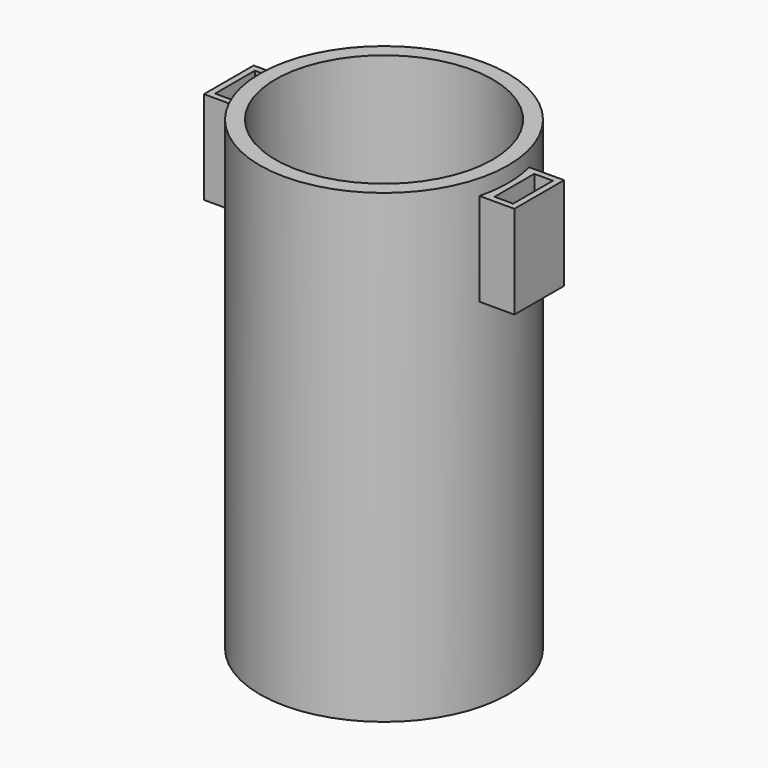
from build123d import *

# Parameters (mm, degrees)
F0_W          = 50.8
F0_H          = 50.8
F1_DEPTH      = 95.25
F3_DEPTH      = 6.35
F5_W          = 3.81
F5_H          = 10.16
F6_DEPTH      = 25.4
F7_T4_DEPTH   = 222.25
F7_T10_DEPTH  = 222.25
F7_T16_DEPTH  = 222.25
F7_T23_DEPTH  = 222.25
F7_T29_DEPTH  = 222.25
F7_T35_DEPTH  = 222.25
F7_T41_DEPTH  = 222.25
F7_T47_DEPTH  = 222.25
F7_T54_DEPTH  = 222.25
F7_T60_DEPTH  = 222.25
F7_T66_DEPTH  = 222.25
F7_T72_DEPTH  = 222.25
F7_T78_DEPTH  = 222.25
F7_T85_DEPTH  = 222.25
F7_T91_DEPTH  = 222.25
F7_T97_DEPTH  = 222.25
F7_T103_DEPTH = 222.25
F7_T109_DEPTH = 222.25
F7_T116_DEPTH = 222.25
F7_T122_DEPTH = 222.25
F8_R          = 22.225
F9_DEPTH      = 88.9


# Not quite as in the source:
# - a fillet or chamfer that OpenCascade refuses, or shapes differently, is made with other operations: its cross-section is extruded or revolved along the edge and cut away or added


with BuildPart() as f1:
    # F0 (on Top) → F1 (new body)
    with BuildSketch(Plane.XY):
        Rectangle(F0_W, F0_H)
    extrude(amount=F1_DEPTH)

    # F2 (on face) → F3 (join)
    with BuildSketch(Plane(origin=(-25.4, 0, 0), x_dir=(0, -1, 0), z_dir=(-1, 0, 0))):
        Polygon((-6.35, 73.025), (6.35, 73.025), (6.35, 92.075), (0, 92.075), (-6.35, 92.075), align=None)
    extrude(amount=F3_DEPTH)

    # F4: F1 across plane


with BuildPart() as f1_1:
    add(f1.part)
    add(f1.part.mirror(Plane.YZ))

    # F5 (on face) → F6 (cut)
    with BuildSketch(Plane.XY.offset(95.25)):
        Polygon((-26.67, -5.08), (-26.67, 0), (-28.575, 0), (-30.48, 0), (-30.48, -5.08), align=None)
        Polygon((-28.575, 0), (-26.67, 0), (-26.67, 5.08), (-30.48, 5.08), (-30.48, 0), align=None)
        with Locations((28.575, 0)):
            Rectangle(F5_W, F5_H)
    extrude(amount=-F6_DEPTH, mode=Mode.SUBTRACT)

    # F7: fillet of radius 25.4 on 4 edges, made by hand


with BuildPart() as f7_tool2:
    # F7_s3 → F7_t4 (new body)
    with BuildSketch(Plane.XY.offset(-63.5)):
        with BuildLine():
            ThreePointArc((0, -25.4), (-17.9605122421, -17.9605122421), (-25.4, 0))
            Line((-25.4, 0), (-25.4, -25.4))
            Line((-25.4, -25.4), (0, -25.4))
        make_face()
    extrude(amount=F7_T4_DEPTH)

    split(bisect_by=Plane.XZ.offset(6.35), keep=Keep.TOP)

    split(bisect_by=Plane.XY.offset(73.025), keep=Keep.BOTTOM)


with BuildPart() as f1_2:
    add(f1_1.part)

    # F7_t1: cut F7_tool2
    add(f7_tool2.part, mode=Mode.SUBTRACT)


with BuildPart() as f7_tool8:
    # F7_s9 → F7_t10 (new body)
    with BuildSketch(Plane.XY.offset(-63.5)):
        with BuildLine():
            ThreePointArc((0, -25.4), (-17.9605122421, -17.9605122421), (-25.4, 0))
            Line((-25.4, 0), (-25.4, -25.4))
            Line((-25.4, -25.4), (0, -25.4))
        make_face()
    extrude(amount=F7_T10_DEPTH)

    split(bisect_by=Plane.XZ.offset(6.35), keep=Keep.BOTTOM)

    split(bisect_by=Plane.XY.offset(73.025), keep=Keep.BOTTOM)


with BuildPart() as f1_3:
    add(f1_2.part)

    # F7_t7: cut F7_tool8
    add(f7_tool8.part, mode=Mode.SUBTRACT)


with BuildPart() as f7_tool14:
    # F7_s15 → F7_t16 (new body)
    with BuildSketch(Plane.XY.offset(-63.5)):
        with BuildLine():
            ThreePointArc((0, -25.4), (-17.9605122421, -17.9605122421), (-25.4, 0))
            Line((-25.4, 0), (-25.4, -25.4))
            Line((-25.4, -25.4), (0, -25.4))
        make_face()
    extrude(amount=F7_T16_DEPTH)

    split(bisect_by=Plane.XY.offset(92.075), keep=Keep.BOTTOM)

    split(bisect_by=Plane.XZ.offset(6.35), keep=Keep.TOP)

    split(bisect_by=Plane.XY.offset(73.025), keep=Keep.TOP)


with BuildPart() as f1_4:
    add(f1_3.part)

    # F7_t13: cut F7_tool14
    add(f7_tool14.part, mode=Mode.SUBTRACT)


with BuildPart() as f7_tool21:
    # F7_s22 → F7_t23 (new body)
    with BuildSketch(Plane.XY.offset(-63.5)):
        with BuildLine():
            ThreePointArc((0, -25.4), (-17.9605122421, -17.9605122421), (-25.4, 0))
            Line((-25.4, 0), (-25.4, -25.4))
            Line((-25.4, -25.4), (0, -25.4))
        make_face()
    extrude(amount=F7_T23_DEPTH)

    split(bisect_by=Plane.XY.offset(92.075), keep=Keep.TOP)

    split(bisect_by=Plane.XZ.offset(6.35), keep=Keep.TOP)


with BuildPart() as f1_5:
    add(f1_4.part)

    # F7_t20: cut F7_tool21
    add(f7_tool21.part, mode=Mode.SUBTRACT)


with BuildPart() as f7_tool27:
    # F7_s28 → F7_t29 (new body)
    with BuildSketch(Plane.XY.offset(-63.5)):
        with BuildLine():
            ThreePointArc((0, -25.4), (-17.9605122421, -17.9605122421), (-25.4, 0))
            Line((-25.4, 0), (-25.4, -25.4))
            Line((-25.4, -25.4), (0, -25.4))
        make_face()
    extrude(amount=F7_T29_DEPTH)

    split(bisect_by=Plane.XY.offset(92.075), keep=Keep.TOP)

    split(bisect_by=Plane.XZ.offset(6.35), keep=Keep.BOTTOM)


with BuildPart() as f1_6:
    add(f1_5.part)

    # F7_t26: cut F7_tool27
    add(f7_tool27.part, mode=Mode.SUBTRACT)


with BuildPart() as f7_tool33:
    # F7_s34 → F7_t35 (new body)
    with BuildSketch(Plane.XY.offset(-63.5)):
        with BuildLine():
            ThreePointArc((0, -25.4), (17.9605122421, -17.9605122421), (25.4, 0))
            Line((25.4, 0), (25.4, -25.4))
            Line((25.4, -25.4), (0, -25.4))
        make_face()
    extrude(amount=F7_T35_DEPTH)

    split(bisect_by=Plane.XY.offset(73.025), keep=Keep.BOTTOM)

    split(bisect_by=Plane.XZ.offset(6.35), keep=Keep.TOP)


with BuildPart() as f1_7:
    add(f1_6.part)

    # F7_t32: cut F7_tool33
    add(f7_tool33.part, mode=Mode.SUBTRACT)


with BuildPart() as f7_tool39:
    # F7_s40 → F7_t41 (new body)
    with BuildSketch(Plane.XY.offset(-63.5)):
        with BuildLine():
            ThreePointArc((0, -25.4), (17.9605122421, -17.9605122421), (25.4, 0))
            Line((25.4, 0), (25.4, -25.4))
            Line((25.4, -25.4), (0, -25.4))
        make_face()
    extrude(amount=F7_T41_DEPTH)

    split(bisect_by=Plane.XY.offset(73.025), keep=Keep.BOTTOM)

    split(bisect_by=Plane.XZ.offset(6.35), keep=Keep.BOTTOM)


with BuildPart() as f1_8:
    add(f1_7.part)

    # F7_t38: cut F7_tool39
    add(f7_tool39.part, mode=Mode.SUBTRACT)


with BuildPart() as f7_tool45:
    # F7_s46 → F7_t47 (new body)
    with BuildSketch(Plane.XY.offset(-63.5)):
        with BuildLine():
            ThreePointArc((0, -25.4), (17.9605122421, -17.9605122421), (25.4, 0))
            Line((25.4, 0), (25.4, -25.4))
            Line((25.4, -25.4), (0, -25.4))
        make_face()
    extrude(amount=F7_T47_DEPTH)

    split(bisect_by=Plane.XY.offset(73.025), keep=Keep.TOP)

    split(bisect_by=Plane.XZ.offset(6.35), keep=Keep.TOP)

    split(bisect_by=Plane.XY.offset(92.075), keep=Keep.BOTTOM)


with BuildPart() as f1_9:
    add(f1_8.part)

    # F7_t44: cut F7_tool45
    add(f7_tool45.part, mode=Mode.SUBTRACT)


with BuildPart() as f7_tool52:
    # F7_s53 → F7_t54 (new body)
    with BuildSketch(Plane.XY.offset(-63.5)):
        with BuildLine():
            ThreePointArc((0, -25.4), (17.9605122421, -17.9605122421), (25.4, 0))
            Line((25.4, 0), (25.4, -25.4))
            Line((25.4, -25.4), (0, -25.4))
        make_face()
    extrude(amount=F7_T54_DEPTH)

    split(bisect_by=Plane.XZ.offset(6.35), keep=Keep.TOP)

    split(bisect_by=Plane.XY.offset(92.075), keep=Keep.TOP)


with BuildPart() as f1_10:
    add(f1_9.part)

    # F7_t51: cut F7_tool52
    add(f7_tool52.part, mode=Mode.SUBTRACT)


with BuildPart() as f7_tool58:
    # F7_s59 → F7_t60 (new body)
    with BuildSketch(Plane.XY.offset(-63.5)):
        with BuildLine():
            ThreePointArc((0, -25.4), (17.9605122421, -17.9605122421), (25.4, 0))
            Line((25.4, 0), (25.4, -25.4))
            Line((25.4, -25.4), (0, -25.4))
        make_face()
    extrude(amount=F7_T60_DEPTH)

    split(bisect_by=Plane.XZ.offset(6.35), keep=Keep.BOTTOM)

    split(bisect_by=Plane.XY.offset(92.075), keep=Keep.TOP)


with BuildPart() as f1_11:
    add(f1_10.part)

    # F7_t57: cut F7_tool58
    add(f7_tool58.part, mode=Mode.SUBTRACT)


with BuildPart() as f7_tool64:
    # F7_s65 → F7_t66 (new body)
    with BuildSketch(Plane.XY.offset(-63.5)):
        with BuildLine():
            ThreePointArc((25.4, 0), (17.9605122421, 17.9605122421), (0, 25.4))
            Line((0, 25.4), (25.4, 25.4))
            Line((25.4, 25.4), (25.4, 0))
        make_face()
    extrude(amount=F7_T66_DEPTH)

    split(bisect_by=Plane.XZ.offset(-6.35), keep=Keep.TOP)

    split(bisect_by=Plane.XY.offset(73.025), keep=Keep.BOTTOM)


with BuildPart() as f1_12:
    add(f1_11.part)

    # F7_t63: cut F7_tool64
    add(f7_tool64.part, mode=Mode.SUBTRACT)


with BuildPart() as f7_tool70:
    # F7_s71 → F7_t72 (new body)
    with BuildSketch(Plane.XY.offset(-63.5)):
        with BuildLine():
            ThreePointArc((25.4, 0), (17.9605122421, 17.9605122421), (0, 25.4))
            Line((0, 25.4), (25.4, 25.4))
            Line((25.4, 25.4), (25.4, 0))
        make_face()
    extrude(amount=F7_T72_DEPTH)

    split(bisect_by=Plane.XZ.offset(-6.35), keep=Keep.BOTTOM)

    split(bisect_by=Plane.XY.offset(73.025), keep=Keep.BOTTOM)


with BuildPart() as f1_13:
    add(f1_12.part)

    # F7_t69: cut F7_tool70
    add(f7_tool70.part, mode=Mode.SUBTRACT)


with BuildPart() as f7_tool76:
    # F7_s77 → F7_t78 (new body)
    with BuildSketch(Plane.XY.offset(-63.5)):
        with BuildLine():
            ThreePointArc((25.4, 0), (17.9605122421, 17.9605122421), (0, 25.4))
            Line((0, 25.4), (25.4, 25.4))
            Line((25.4, 25.4), (25.4, 0))
        make_face()
    extrude(amount=F7_T78_DEPTH)

    split(bisect_by=Plane.XZ.offset(-6.35), keep=Keep.BOTTOM)

    split(bisect_by=Plane.XY.offset(73.025), keep=Keep.TOP)

    split(bisect_by=Plane.XY.offset(92.075), keep=Keep.BOTTOM)


with BuildPart() as f1_14:
    add(f1_13.part)

    # F7_t75: cut F7_tool76
    add(f7_tool76.part, mode=Mode.SUBTRACT)


with BuildPart() as f7_tool83:
    # F7_s84 → F7_t85 (new body)
    with BuildSketch(Plane.XY.offset(-63.5)):
        with BuildLine():
            ThreePointArc((25.4, 0), (17.9605122421, 17.9605122421), (0, 25.4))
            Line((0, 25.4), (25.4, 25.4))
            Line((25.4, 25.4), (25.4, 0))
        make_face()
    extrude(amount=F7_T85_DEPTH)

    split(bisect_by=Plane.XZ.offset(-6.35), keep=Keep.TOP)

    split(bisect_by=Plane.XY.offset(92.075), keep=Keep.TOP)


with BuildPart() as f1_15:
    add(f1_14.part)

    # F7_t82: cut F7_tool83
    add(f7_tool83.part, mode=Mode.SUBTRACT)


with BuildPart() as f7_tool89:
    # F7_s90 → F7_t91 (new body)
    with BuildSketch(Plane.XY.offset(-63.5)):
        with BuildLine():
            ThreePointArc((25.4, 0), (17.9605122421, 17.9605122421), (0, 25.4))
            Line((0, 25.4), (25.4, 25.4))
            Line((25.4, 25.4), (25.4, 0))
        make_face()
    extrude(amount=F7_T91_DEPTH)

    split(bisect_by=Plane.XZ.offset(-6.35), keep=Keep.BOTTOM)

    split(bisect_by=Plane.XY.offset(92.075), keep=Keep.TOP)


with BuildPart() as f1_16:
    add(f1_15.part)

    # F7_t88: cut F7_tool89
    add(f7_tool89.part, mode=Mode.SUBTRACT)


with BuildPart() as f7_tool95:
    # F7_s96 → F7_t97 (new body)
    with BuildSketch(Plane.XY.offset(-63.5)):
        with BuildLine():
            ThreePointArc((-25.4, 0), (-17.9605122421, 17.9605122421), (0, 25.4))
            Line((0, 25.4), (-25.4, 25.4))
            Line((-25.4, 25.4), (-25.4, 0))
        make_face()
    extrude(amount=F7_T97_DEPTH)

    split(bisect_by=Plane.XZ.offset(-6.35), keep=Keep.TOP)

    split(bisect_by=Plane.XY.offset(73.025), keep=Keep.BOTTOM)


with BuildPart() as f1_17:
    add(f1_16.part)

    # F7_t94: cut F7_tool95
    add(f7_tool95.part, mode=Mode.SUBTRACT)


with BuildPart() as f7_tool101:
    # F7_s102 → F7_t103 (new body)
    with BuildSketch(Plane.XY.offset(-63.5)):
        with BuildLine():
            ThreePointArc((-25.4, 0), (-17.9605122421, 17.9605122421), (0, 25.4))
            Line((0, 25.4), (-25.4, 25.4))
            Line((-25.4, 25.4), (-25.4, 0))
        make_face()
    extrude(amount=F7_T103_DEPTH)

    split(bisect_by=Plane.XZ.offset(-6.35), keep=Keep.BOTTOM)

    split(bisect_by=Plane.XY.offset(73.025), keep=Keep.BOTTOM)


with BuildPart() as f1_18:
    add(f1_17.part)

    # F7_t100: cut F7_tool101
    add(f7_tool101.part, mode=Mode.SUBTRACT)


with BuildPart() as f7_tool107:
    # F7_s108 → F7_t109 (new body)
    with BuildSketch(Plane.XY.offset(-63.5)):
        with BuildLine():
            ThreePointArc((-25.4, 0), (-17.9605122421, 17.9605122421), (0, 25.4))
            Line((0, 25.4), (-25.4, 25.4))
            Line((-25.4, 25.4), (-25.4, 0))
        make_face()
    extrude(amount=F7_T109_DEPTH)

    split(bisect_by=Plane.XZ.offset(-6.35), keep=Keep.BOTTOM)

    split(bisect_by=Plane.XY.offset(92.075), keep=Keep.BOTTOM)

    split(bisect_by=Plane.XY.offset(73.025), keep=Keep.TOP)


with BuildPart() as f1_19:
    add(f1_18.part)

    # F7_t106: cut F7_tool107
    add(f7_tool107.part, mode=Mode.SUBTRACT)


with BuildPart() as f7_tool114:
    # F7_s115 → F7_t116 (new body)
    with BuildSketch(Plane.XY.offset(-63.5)):
        with BuildLine():
            ThreePointArc((-25.4, 0), (-17.9605122421, 17.9605122421), (0, 25.4))
            Line((0, 25.4), (-25.4, 25.4))
            Line((-25.4, 25.4), (-25.4, 0))
        make_face()
    extrude(amount=F7_T116_DEPTH)

    split(bisect_by=Plane.XZ.offset(-6.35), keep=Keep.TOP)

    split(bisect_by=Plane.XY.offset(92.075), keep=Keep.TOP)


with BuildPart() as f1_20:
    add(f1_19.part)

    # F7_t113: cut F7_tool114
    add(f7_tool114.part, mode=Mode.SUBTRACT)


with BuildPart() as f7_tool120:
    # F7_s121 → F7_t122 (new body)
    with BuildSketch(Plane.XY.offset(-63.5)):
        with BuildLine():
            ThreePointArc((-25.4, 0), (-17.9605122421, 17.9605122421), (0, 25.4))
            Line((0, 25.4), (-25.4, 25.4))
            Line((-25.4, 25.4), (-25.4, 0))
        make_face()
    extrude(amount=F7_T122_DEPTH)

    split(bisect_by=Plane.XZ.offset(-6.35), keep=Keep.BOTTOM)

    split(bisect_by=Plane.XY.offset(92.075), keep=Keep.TOP)


with BuildPart() as f1_21:
    add(f1_20.part)

    # F7_t119: cut F7_tool120
    add(f7_tool120.part, mode=Mode.SUBTRACT)

    # F8 (on face) → F9 (cut)
    with BuildSketch(Plane.XY.offset(95.25)):
        Circle(F8_R)
    extrude(amount=-F9_DEPTH, mode=Mode.SUBTRACT)


solid = f1_21.part
